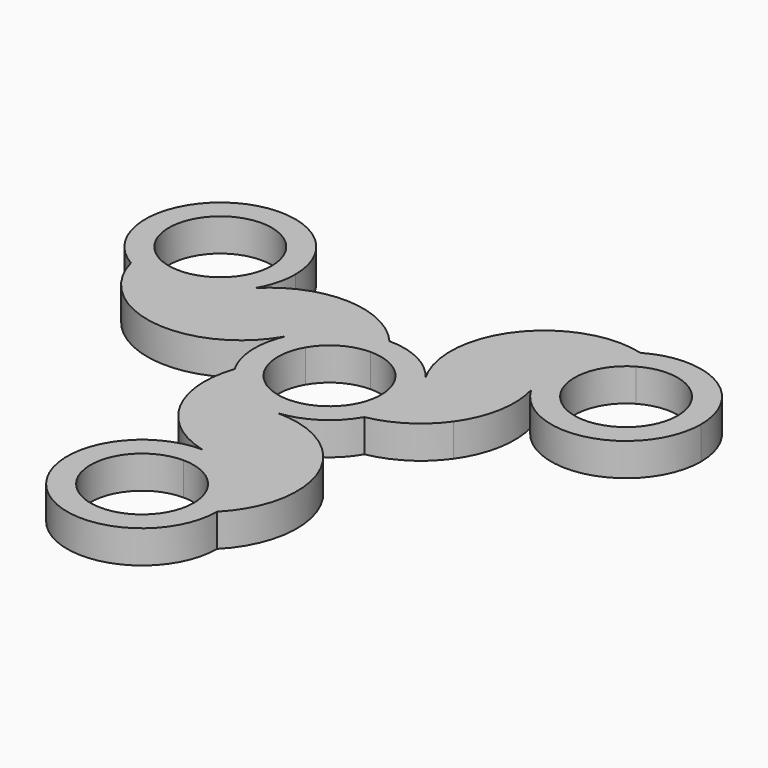
from build123d import *

# Parameters (mm, degrees)
F1_DEPTH = 7


# Not quite as in the source:
# - a feature names something its author has since deleted; it is built from what else it names


with BuildPart() as f1:
    # F0 (on Top) → F1 (new body)
    with BuildSketch(Plane.XY):
        with BuildLine():
            Line((16, 0), (11, 0))
            ThreePointArc((11, 0), (10.6251840892, -2.8470094961), (9.5262794416, -5.5))
            Line((9.5262794416, -5.5), (13.8564064606, -8))
            ThreePointArc((13.8564064606, -8), (15.4548132206, -4.1411047216), (16, 0))
        make_face()
        with BuildLine():
            ThreePointArc((9.5262794416, 5.5), (10.6251840892, 2.8470094961), (11, 0))
            Line((11, 0), (16, 0))
            ThreePointArc((16, 0), (15.4548132206, 4.1411047216), (13.8564064606, 8))
            Line((13.8564064606, 8), (9.5262794416, 5.5))
        make_face()
        with BuildLine():
            ThreePointArc((0, 11), (5.5, 9.5262794416), (9.5262794416, 5.5))
            Line((9.5262794416, 5.5), (13.8564064606, 8))
            ThreePointArc((13.8564064606, 8), (13.409185793, 8.6628012124), (12.9888150126, 9.3429483874))
            ThreePointArc((12.9888150126, 9.3429483874), (7.2976991512, 14.2388056767), (0, 16))
            Line((0, 16), (0, 11))
        make_face()
        with BuildLine():
            Line((13.8564064606, -8), (9.5262794416, -5.5))
            ThreePointArc((9.5262794416, -5.5), (5.5, -9.5262794416), (0, -11))
            Line((0, -11), (0, -16))
            ThreePointArc((0, -16), (0.7976130214, -15.944096147), (1.5968231434, -15.9201179596))
            ThreePointArc((1.5968231434, -15.9201179596), (8.68231786, -13.4393956924), (13.8564064606, -8))
        make_face()
        with BuildLine():
            Line((26.4227403385, 0), (16, 0))
            ThreePointArc((16, 0), (15.4548132206, -4.1411047216), (13.8564064606, -8))
            ThreePointArc((13.8564064606, -8), (20.912199664, -5.2136349503), (26.4227403385, 0))
        make_face()
        with BuildLine():
            ThreePointArc((13.8564064606, 8), (15.4548132206, 4.1411047216), (16, 0))
            Line((16, 0), (26.4227403385, 0))
            ThreePointArc((26.4227403385, 0), (29.8628617611, 8.1570672633), (29.4448637287, 17))
            Line((29.4448637287, 17), (13.8564064606, 8))
        make_face()
        with BuildLine():
            ThreePointArc((-9.5262794416, 5.5), (-5.5, 9.5262794416), (0, 11))
            Line((0, 11), (0, 16))
            ThreePointArc((0, 16), (-8, 13.8564064606), (-13.8564064606, 8))
            Line((-13.8564064606, 8), (-9.5262794416, 5.5))
        make_face()
        with BuildLine():
            ThreePointArc((12.9888150126, 9.3429483874), (13.409185793, 8.6628012124), (13.8564064606, 8))
            ThreePointArc((13.8564064606, 8), (13.4393956924, 8.68231786), (12.9888150126, 9.3429483874))
        make_face()
        with BuildLine():
            ThreePointArc((12.9888150126, 9.3429483874), (13.4393956924, 8.68231786), (13.8564064606, 8))
            Line((13.8564064606, 8), (29.4448637287, 17))
            ThreePointArc((29.4448637287, 17), (27.8464569686, 29.1411047216), (35.3012701892, 38.8564064606))
            ThreePointArc((35.3012701892, 38.8564064606), (14.2545680685, 31.576970296), (12.9888150126, 9.3429483874))
        make_face()
        with BuildLine():
            Line((0, -16), (0, -11))
            ThreePointArc((0, -11), (-5.5, -9.5262794416), (-9.5262794416, -5.5))
            Line((-9.5262794416, -5.5), (-13.8564064606, -8))
            ThreePointArc((-13.8564064606, -8), (-8, -13.8564064606), (0, -16))
        make_face()
        with BuildLine():
            ThreePointArc((-9.5262794416, -5.5), (-11, 0), (-9.5262794416, 5.5))
            Line((-9.5262794416, 5.5), (-13.8564064606, 8))
            ThreePointArc((-13.8564064606, 8), (-14.2067988144, 7.2812949346), (-14.585638156, 6.5771695722))
            ThreePointArc((-14.585638156, 6.5771695722), (-15.9800170112, -0.7994099843), (-13.8564064606, -8))
            Line((-13.8564064606, -8), (-9.5262794416, -5.5))
        make_face()
        with BuildLine():
            ThreePointArc((-13.8564064606, 8), (-8, 13.8564064606), (0, 16))
            ThreePointArc((0, 16), (-14.5027493597, 22.9685214121), (-29.4448637287, 17))
            Line((-29.4448637287, 17), (-13.8564064606, 8))
        make_face()
        with BuildLine():
            ThreePointArc((35.3012701892, 38.8564064606), (27.8464569686, 29.1411047216), (29.4448637287, 17))
            Line((29.4448637287, 17), (33.7749907476, 19.5))
            ThreePointArc((33.7749907476, 19.5), (32.6760861, 27.8470094961), (37.8012701892, 34.5262794416))
            Line((37.8012701892, 34.5262794416), (35.3012701892, 38.8564064606))
        make_face()
        with BuildLine():
            Line((33.7749907476, 19.5), (29.4448637287, 17))
            ThreePointArc((29.4448637287, 17), (47.4423749109, 9.5451867794), (59.3012701892, 25))
            ThreePointArc((59.3012701892, 25), (51.3012701892, 38.8564064606), (35.3012701892, 38.8564064606))
            Line((35.3012701892, 38.8564064606), (37.8012701892, 34.5262794416))
            ThreePointArc((37.8012701892, 34.5262794416), (48.8012701892, 34.5262794416), (54.3012701892, 25))
            ThreePointArc((54.3012701892, 25), (46.1482796853, 14.3748159108), (33.7749907476, 19.5))
        make_face()
        with BuildLine():
            Line((0, -34), (0, -16))
            ThreePointArc((0, -16), (-8, -13.8564064606), (-13.8564064606, -8))
            ThreePointArc((-13.8564064606, -8), (-12.6399483504, -24.0440100763), (0, -34))
        make_face()
        with BuildLine():
            ThreePointArc((1.5968231434, -15.9201179596), (0.7976130214, -15.944096147), (0, -16))
            ThreePointArc((0, -16), (0.7994099843, -15.9800170112), (1.5968231434, -15.9201179596))
        make_face()
        with BuildLine():
            ThreePointArc((1.5968231434, -15.9201179596), (0.7994099843, -15.9800170112), (0, -16))
            Line((0, -16), (0, -34))
            ThreePointArc((0, -34), (11.313708499, -38.686291501), (16, -50))
            ThreePointArc((16, -50), (20.2191744167, -28.1333032153), (1.5968231434, -15.9201179596))
        make_face()
        with BuildLine():
            ThreePointArc((-14.585638156, 6.5771695722), (-14.2067988144, 7.2812949346), (-13.8564064606, 8))
            ThreePointArc((-13.8564064606, 8), (-14.2388056767, 7.2976991512), (-14.585638156, 6.5771695722))
        make_face()
        with BuildLine():
            ThreePointArc((-14.585638156, 6.5771695722), (-14.2388056767, 7.2976991512), (-13.8564064606, 8))
            Line((-13.8564064606, 8), (-29.4448637287, 17))
            ThreePointArc((-29.4448637287, 17), (-39.1601654676, 9.5451867794), (-51.3012701892, 11.1435935394))
            ThreePointArc((-51.3012701892, 11.1435935394), (-34.4737424851, -3.4436670807), (-14.585638156, 6.5771695722))
        make_face()
        with BuildLine():
            ThreePointArc((-51.3012701892, 11.1435935394), (-39.1601654676, 9.5451867794), (-29.4448637287, 17))
            Line((-29.4448637287, 17), (-33.7749907476, 19.5))
            ThreePointArc((-33.7749907476, 19.5), (-40.4542606931, 14.3748159108), (-48.8012701892, 15.4737205584))
            Line((-48.8012701892, 15.4737205584), (-51.3012701892, 11.1435935394))
        make_face()
        with BuildLine():
            Line((-33.7749907476, 19.5), (-29.4448637287, 17))
            ThreePointArc((-29.4448637287, 17), (-27.8464569686, 20.8588952784), (-27.3012701892, 25))
            ThreePointArc((-27.3012701892, 25), (-51.3012701892, 38.8564064606), (-51.3012701892, 11.1435935394))
            Line((-51.3012701892, 11.1435935394), (-48.8012701892, 15.4737205584))
            ThreePointArc((-48.8012701892, 15.4737205584), (-48.8012701892, 34.5262794416), (-32.3012701892, 25))
            ThreePointArc((-32.3012701892, 25), (-32.6760861, 22.1529905039), (-33.7749907476, 19.5))
        make_face()
        with BuildLine():
            ThreePointArc((16, -50), (11.313708499, -38.686291501), (0, -34))
            Line((0, -34), (0, -39))
            ThreePointArc((0, -39), (7.7781745931, -42.2218254069), (11, -50))
            Line((11, -50), (16, -50))
        make_face()
        with BuildLine():
            Line((0, -39), (0, -34))
            ThreePointArc((0, -34), (-11.313708499, -61.313708499), (16, -50))
            Line((16, -50), (11, -50))
            ThreePointArc((11, -50), (-7.7781745931, -57.7781745931), (0, -39))
        make_face()
    extrude(amount=F1_DEPTH)


solid = f1.part
